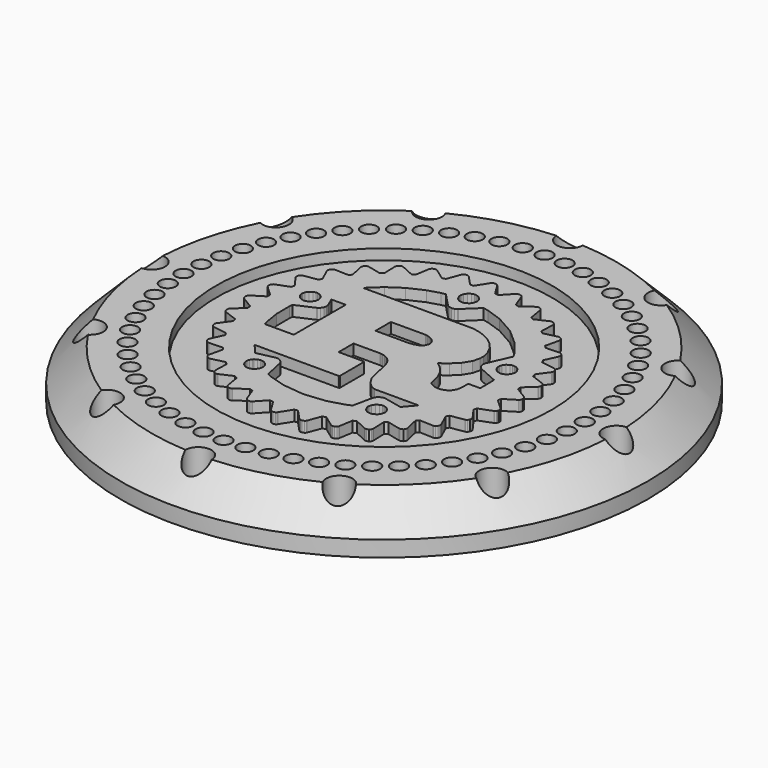
from build123d import *

# Parameters (mm, degrees)
F0_R      = 25
F1_DEPTH  = 3
F2_R      = 0.75
F3_DEPTH  = 3
F4_R      = 1.25
F5_DEPTH  = 3
F7_R      = 15.9136389896
F8_DEPTH  = 1
F10_DEPTH = 1
F11_R     = 25
F11_R_2   = 23
F12_DEPTH = 1.5


# Not quite as in the source:
# - a fillet or chamfer that OpenCascade refuses, or shapes differently, is made with other operations: its cross-section is extruded or revolved along the edge and cut away or added


with BuildPart() as f1:
    # F0 (on Top) → F1 (new body)
    with BuildSketch(Plane.XY):
        Circle(F0_R)
    extrude(amount=F1_DEPTH)

    # F2 (on face) → F3 (cut)
    with BuildSketch(Plane.XY.offset(3)):
        with Locations((0, 19)):
            Circle(F2_R)
        with Locations((-1.9860408021, 18.895916012)):
            Circle(F2_R)
        with Locations((-3.9503221255, 18.5848044139)):
            Circle(F2_R)
        with Locations((-5.8713228931, 18.0700738096)):
            Circle(F2_R)
        with Locations((-7.7279962184, 17.3573636952)):
            Circle(F2_R)
        with Locations((-9.5, 16.4544826719)):
            Circle(F2_R)
        with Locations((-11.1679197936, 15.3713228931)):
            Circle(F2_R)
        with Locations((-12.7134815208, 14.1197516841)):
            Circle(F2_R)
        with Locations((-14.1197516841, 12.7134815208)):
            Circle(F2_R)
        with Locations((-15.3713228931, 11.1679197936)):
            Circle(F2_R)
        with Locations((-16.4544826719, 9.5)):
            Circle(F2_R)
        with Locations((-17.3573636952, 7.7279962184)):
            Circle(F2_R)
        with Locations((-18.0700738096, 5.8713228931)):
            Circle(F2_R)
        with Locations((-18.5848044139, 3.9503221255)):
            Circle(F2_R)
        with Locations((-18.895916012, 1.9860408021)):
            Circle(F2_R)
        with Locations((-19, 0)):
            Circle(F2_R)
        with Locations((-18.895916012, -1.9860408021)):
            Circle(F2_R)
        with Locations((-18.5848044139, -3.9503221255)):
            Circle(F2_R)
        with Locations((-18.0700738096, -5.8713228931)):
            Circle(F2_R)
        with Locations((-17.3573636952, -7.7279962184)):
            Circle(F2_R)
        with Locations((-16.4544826719, -9.5)):
            Circle(F2_R)
        with Locations((-15.3713228931, -11.1679197936)):
            Circle(F2_R)
        with Locations((-14.1197516841, -12.7134815208)):
            Circle(F2_R)
        with Locations((-12.7134815208, -14.1197516841)):
            Circle(F2_R)
        with Locations((-11.1679197936, -15.3713228931)):
            Circle(F2_R)
        with Locations((-9.5, -16.4544826719)):
            Circle(F2_R)
        with Locations((-7.7279962184, -17.3573636952)):
            Circle(F2_R)
        with Locations((-5.8713228931, -18.0700738096)):
            Circle(F2_R)
        with Locations((-3.9503221255, -18.5848044139)):
            Circle(F2_R)
        with Locations((-1.9860408021, -18.895916012)):
            Circle(F2_R)
        with Locations((0, -19)):
            Circle(F2_R)
        with Locations((1.9860408021, -18.895916012)):
            Circle(F2_R)
        with Locations((3.9503221255, -18.5848044139)):
            Circle(F2_R)
        with Locations((5.8713228931, -18.0700738096)):
            Circle(F2_R)
        with Locations((7.7279962184, -17.3573636952)):
            Circle(F2_R)
        with Locations((9.5, -16.4544826719)):
            Circle(F2_R)
        with Locations((11.1679197936, -15.3713228931)):
            Circle(F2_R)
        with Locations((12.7134815208, -14.1197516841)):
            Circle(F2_R)
        with Locations((14.1197516841, -12.7134815208)):
            Circle(F2_R)
        with Locations((15.3713228931, -11.1679197936)):
            Circle(F2_R)
        with Locations((16.4544826719, -9.5)):
            Circle(F2_R)
        with Locations((17.3573636952, -7.7279962184)):
            Circle(F2_R)
        with Locations((18.0700738096, -5.8713228931)):
            Circle(F2_R)
        with Locations((18.5848044139, -3.9503221255)):
            Circle(F2_R)
        with Locations((18.895916012, -1.9860408021)):
            Circle(F2_R)
        with Locations((19, 0)):
            Circle(F2_R)
        with Locations((18.895916012, 1.9860408021)):
            Circle(F2_R)
        with Locations((18.5848044139, 3.9503221255)):
            Circle(F2_R)
        with Locations((18.0700738096, 5.8713228931)):
            Circle(F2_R)
        with Locations((17.3573636952, 7.7279962184)):
            Circle(F2_R)
        with Locations((16.4544826719, 9.5)):
            Circle(F2_R)
        with Locations((15.3713228931, 11.1679197936)):
            Circle(F2_R)
        with Locations((14.1197516841, 12.7134815208)):
            Circle(F2_R)
        with Locations((12.7134815208, 14.1197516841)):
            Circle(F2_R)
        with Locations((11.1679197936, 15.3713228931)):
            Circle(F2_R)
        with Locations((9.5, 16.4544826719)):
            Circle(F2_R)
        with Locations((7.7279962184, 17.3573636952)):
            Circle(F2_R)
        with Locations((5.8713228931, 18.0700738096)):
            Circle(F2_R)
        with Locations((3.9503221255, 18.5848044139)):
            Circle(F2_R)
        with Locations((1.9860408021, 18.895916012)):
            Circle(F2_R)
    extrude(amount=-F3_DEPTH, mode=Mode.SUBTRACT)

    # F4 (on face) → F5 (cut)
    with BuildSketch(Plane.XY.offset(3)):
        with Locations((0, 22)):
            Circle(F4_R)
        with Locations((-11, 19.0525588833)):
            Circle(F4_R)
        with Locations((-19.0525588833, 11)):
            Circle(F4_R)
        with Locations((-22, 0)):
            Circle(F4_R)
        with Locations((-19.0525588833, -11)):
            Circle(F4_R)
        with Locations((-11, -19.0525588833)):
            Circle(F4_R)
        with Locations((0, -22)):
            Circle(F4_R)
        with Locations((11, -19.0525588833)):
            Circle(F4_R)
        with Locations((19.0525588833, -11)):
            Circle(F4_R)
        with Locations((22, 0)):
            Circle(F4_R)
        with Locations((19.0525588833, 11)):
            Circle(F4_R)
        with Locations((11, 19.0525588833)):
            Circle(F4_R)
    extrude(amount=-F5_DEPTH, mode=Mode.SUBTRACT)

    # F6: chamfer of 3 on 1 edges, made by hand

    # F6_s1 → F6_t2 (revolve, cut)
    with BuildSketch(Plane.XZ):
        Polygon((25, 0), (22, 3), (25, 3), align=None)
    revolve(axis=Axis((0, 0, 3), (0, 0, 1)), mode=Mode.SUBTRACT)

    # F7 (on face) → F8 (cut)
    with BuildSketch(Plane.XY.offset(3)):
        Circle(F7_R)
    extrude(amount=-F8_DEPTH, mode=Mode.SUBTRACT)

    # F9 (on face) → F10 (join)
    with BuildSketch(Plane.XY.offset(2)):
        Polygon((12.98642, 0.32225), (11.88072, 1.00693), (11.84932, 1.32865), (12.79912, 2.21461), (12.83232, 2.24554), (12.89522, 2.37737), (12.90122, 2.56567), (12.82412, 2.73707), (12.71512, 2.83417), (12.67332, 2.84937), (11.45912, 3.30347), (11.36372, 3.61707), (12.12162, 4.66957), (12.14762, 4.70647), (12.18402, 4.84757), (12.15302, 5.03307), (12.04342, 5.18607), (11.91822, 5.26037), (11.87362, 5.26747), (10.59332, 5.47577), (10.43912, 5.76337), (10.97732, 6.94447), (10.99582, 6.98557), (11.00452, 7.13157), (10.93832, 7.30797), (10.80112, 7.43697), (10.66332, 7.48417), (10.61822, 7.48267), (9.31832, 7.43697), (9.11322, 7.68657), (9.41162, 8.95237), (9.42192, 8.99687), (9.40132, 9.14117), (9.30152, 9.30057), (9.14252, 9.40047), (8.99822, 9.42057), (8.95432, 9.41017), (7.68862, 9.11187), (7.43902, 9.31697), (7.48452, 10.61687), (7.48622, 10.66237), (7.43792, 10.79967), (7.30872, 10.93647), (7.13302, 11.00367), (6.98702, 10.99547), (6.94632, 10.97657), (5.76522, 10.43787), (5.47772, 10.59237), (5.26882, 11.87337), (5.26182, 11.91787), (5.18742, 12.04307), (5.03442, 12.15227), (4.84892, 12.18367), (4.70782, 12.14727), (4.67152, 12.12077), (3.61842, 11.36337), (3.30542, 11.45787), (2.85132, 12.67257), (2.83552, 12.71537), (2.73842, 12.82437), (2.56647, 12.90147), (2.3782, 12.89607), (2.24745, 12.83257), (2.21654, 12.79947), (1.33058, 11.84837), (1.00884, 11.87987), (0.32418, 12.98557), (0.3003, 13.02407), (0.18365, 13.11197), (0.00027, 13.15377), (-0.1831, 13.11197), (-0.2992, 13.02407), (-0.32253, 12.98557), (-1.00667, 11.87987), (-1.32894, 11.84837), (-2.21544, 12.79947), (-2.24637, 12.83257), (-2.37766, 12.89607), (-2.56591, 12.90147), (-2.73789, 12.82437), (-2.83446, 12.71537), (-2.8502, 12.67257), (-3.3043, 11.45787), (-3.61734, 11.36337), (-4.66987, 12.12077), (-4.70675, 12.14727), (-4.84781, 12.18427), (-5.03337, 12.15287), (-5.18744, 12.04307), (-5.26123, 11.91787), (-5.26828, 11.87337), (-5.47662, 10.59237), (-5.76416, 10.43787), (-6.94525, 10.97657), (-6.98649, 10.99547), (-7.13243, 11.00367), (-7.30821, 10.93697), (-7.43733, 10.79967), (-7.48508, 10.66237), (-7.48345, 10.61687), (-7.43787, 9.31697), (-7.68744, 9.11187), (-8.95317, 9.41017), (-8.99766, 9.42057), (-9.14198, 9.40047), (-9.30148, 9.30007), (-9.40185, 9.14117), (-9.42138, 8.99687), (-9.41107, 8.95237), (-9.11323, 7.68657), (-9.31775, 7.43697), (-10.61767, 7.48267), (-10.66324, 7.48417), (-10.79996, 7.43607), (-10.93669, 7.30687), (-11.00395, 7.13107), (-10.99582, 6.98557), (-10.97682, 6.94447), (-10.43863, 5.76337), (-10.59271, 5.47577), (-11.87364, 5.26747), (-11.91867, 5.26037), (-12.04399, 5.18667), (-12.15251, 5.03307), (-12.18396, 4.84757), (-12.14762, 4.70647), (-12.12103, 4.66957), (-11.36366, 3.61707), (-11.4586, 3.30347), (-12.67334, 2.84937), (-12.71566, 2.83367), (-12.82416, 2.73707), (-12.9012, 2.56567), (-12.89577, 2.37737), (-12.8323, 2.24554), (-12.7992, 2.21461), (-11.84923, 1.32865), (-11.88069, 1.00693), (-12.98584, 0.32225), (-13.02435, 0.29891), (-13.11224, 0.18228), (-13.15402, -0.0011), (-13.11224, -0.18447), (-13.02435, -0.30059), (-12.98584, -0.32445), (-11.88069, -1.00859), (-11.84923, -1.33085), (-12.7992, -2.21735), (-12.8323, -2.24774), (-12.89577, -2.37903), (-12.9012, -2.56675), (-12.82416, -2.73872), (-12.71566, -2.83585), (-12.67334, -2.85157), (-11.4586, -3.30568), (-11.36366, -3.61927), (-12.12103, -4.67178), (-12.14762, -4.70813), (-12.18396, -4.84974), (-12.15251, -5.03528), (-12.04345, -5.18828), (-11.91813, -5.2626), (-11.8731, -5.26966), (-10.59271, -5.47799), (-10.43863, -5.76607), (-10.97682, -6.94663), (-10.99582, -6.98732), (-11.0045, -7.13326), (-10.93723, -7.30904), (-10.79996, -7.43871), (-10.6627, -7.48645), (-10.61767, -7.48482), (-9.3183, -7.43925), (-9.11323, -7.68882), (-9.41107, -8.95509), (-9.42138, -8.9985), (-9.40185, -9.14281), (-9.30148, -9.30232), (-9.14198, -9.4016), (-8.99766, -9.42221), (-8.95317, -9.41191), (-7.68744, -9.11352), (-7.43787, -9.3186), (-7.48345, -10.6185), (-7.48508, -10.66353), (-7.43733, -10.80079), (-7.30821, -10.93752), (-7.13243, -11.00425), (-6.98649, -10.99611), (-6.94525, -10.97767), (-5.76416, -10.43947), (-5.47662, -10.59409), (-5.26828, -11.87393), (-5.26123, -11.91842), (-5.18744, -12.04374), (-5.03337, -12.15279), (-4.84781, -12.18427), (-4.70675, -12.14791), (-4.66987, -12.12186), (-3.61789, -11.36395), (-3.3043, -11.45943), (-2.8502, -12.67363), (-2.83446, -12.71541), (-2.73789, -12.82391), (-2.56591, -12.90095), (-2.3782, -12.89553), (-2.24691, -12.83259), (-2.21598, -12.7995), (-1.32948, -11.84952), (-1.00721, -11.88153), (-0.32253, -12.98721), (-0.2992, -13.0252), (-0.1831, -13.112), (0.00027, -13.15377), (0.18365, -13.11254), (0.3003, -13.0252), (0.32418, -12.98721), (1.0083, -11.88153), (1.33058, -11.84952), (2.21654, -12.7995), (2.24691, -12.83204), (2.3782, -12.89553), (2.56647, -12.90095), (2.73842, -12.82391), (2.83552, -12.71541), (2.85132, -12.67363), (3.30542, -11.45943), (3.61842, -11.36395), (4.67092, -12.12186), (4.70732, -12.14791), (4.84832, -12.18427), (5.03392, -12.15279), (5.18742, -12.04374), (5.26122, -11.91842), (5.26882, -11.87393), (5.47772, -10.59409), (5.76522, -10.43947), (6.94632, -10.97767), (6.98702, -10.99611), (7.13252, -11.00479), (7.30872, -10.93806), (7.43732, -10.80079), (7.48572, -10.66353), (7.48402, -10.6185), (7.43902, -9.3186), (7.68802, -9.11352), (8.95372, -9.41191), (8.99762, -9.42221), (9.14192, -9.4016), (9.30152, -9.30232), (9.40132, -9.14281), (9.42142, -8.9985), (9.41162, -8.95509), (9.11322, -7.68882), (9.31832, -7.43925), (10.61762, -7.48482), (10.66272, -7.48645), (10.80002, -7.43871), (10.93722, -7.30904), (11.00452, -7.13326), (10.99582, -6.98732), (10.97732, -6.94663), (10.43912, -5.76607), (10.59272, -5.47799), (11.87362, -5.26966), (11.91822, -5.2626), (12.04342, -5.18828), (12.15252, -5.03528), (12.18402, -4.84974), (12.14702, -4.70813), (12.12112, -4.67178), (11.36372, -3.61927), (11.45862, -3.30568), (12.67332, -2.85157), (12.71572, -2.83585), (12.82412, -2.73872), (12.90122, -2.56675), (12.89522, -2.37903), (12.83182, -2.24774), (12.79912, -2.21735), (11.84932, -1.33085), (11.88072, -1.00859), (12.98582, -0.32445), (13.02392, -0.30059), (13.11162, -0.18447), (13.15402, -0.0011), (13.11222, 0.18228), (13.02442, 0.29891), align=None)
        Polygon((-6.61593, -8.12068), (-6.61593, -8.04472), (-6.61593, -7.96985), (-6.5568, -7.74524), (-6.42388, -7.52769), (-6.38699, -7.49134), (-6.35064, -7.45444), (-6.13362, -7.32152), (-5.90901, -7.26239), (-5.83414, -7.26239), (-5.75981, -7.26239), (-5.5352, -7.32152), (-5.31819, -7.45444), (-5.2813, -7.49134), (-5.24495, -7.52769), (-5.11203, -7.74524), (-5.05235, -7.96985), (-5.05235, -8.04472), (-5.05235, -8.12068), (-5.1142, -8.34854), (-5.2813, -8.59756), (-5.53032, -8.76466), (-5.75819, -8.82651), (-5.83414, -8.82651), (-5.91064, -8.82651), (-6.1385, -8.76466), (-6.38699, -8.59756), (-6.55463, -8.34854), align=None, mode=Mode.SUBTRACT)
        Polygon((4.96992, -8.15703), (4.96992, -8.08107), (4.96992, -8.00457), (5.03122, -7.77671), (5.19882, -7.52823), (5.44732, -7.36058), (5.67522, -7.29928), (5.75172, -7.29928), (5.82762, -7.29928), (6.05552, -7.36058), (6.30452, -7.52823), (6.47222, -7.77671), (6.53402, -8.00457), (6.53402, -8.08107), (6.53402, -8.15703), (6.47222, -8.38489), (6.30452, -8.63337), (6.05552, -8.80047), (5.82762, -8.86232), (5.75172, -8.86232), (5.67522, -8.86232), (5.44732, -8.80047), (5.19882, -8.63337), (5.03122, -8.38489), align=None, mode=Mode.SUBTRACT)
        Polygon((6.86552, -6.66343), (5.21192, -6.30753), (5.14352, -6.29288), (4.92812, -6.30372), (4.67472, -6.40572), (4.47782, -6.59561), (4.37912, -6.78767), (4.36492, -6.85603), (3.97272, -8.68762), (3.50182, -8.9003), (1.99788, -9.33596), (-0.04584, -9.54538), (-2.08794, -9.31588), (-3.58751, -8.86666), (-4.05571, -8.6491), (-4.44796, -6.81751), (-4.46262, -6.74969), (-4.56135, -6.55763), (-4.7583, -6.36775), (-5.01166, -6.26575), (-5.22705, -6.25491), (-5.29432, -6.26954), (-6.91162, -6.61677), (-6.98703, -6.53919), (-7.68364, -5.71779), (-7.74766, -5.63099), (0.12018, -5.63099), (0.14676, -5.63099), (0.22759, -5.61254), (0.26883, -5.5534), (0.26883, -5.53386), (0.26883, -2.75121), (0.26883, -2.73114), (0.22759, -2.672), (0.14676, -2.6541), (0.12018, -2.6541), (-2.18071, -2.6541), (-2.18071, -0.88977), (0.3079, -0.88977), (0.33719, -0.88977), (0.42562, -0.89465), (0.59815, -0.91961), (0.80865, -0.97657), (1.03977, -1.07965), (1.27523, -1.24188), (1.49768, -1.47679), (1.69081, -1.79743), (1.81126, -2.10939), (1.83838, -2.21681), (1.8628, -2.31393), (1.9317, -2.64488), (2.05161, -3.2384), (2.18127, -3.83465), (2.26536, -4.17047), (2.3028, -4.27193), (2.33697, -4.37664), (2.49213, -4.67559), (2.81332, -5.12154), (3.22732, -5.48234), (3.57772, -5.63099), (3.69492, -5.63099), (7.75692, -5.63099), (7.68862, -5.72213), (6.94582, -6.58259), align=None, mode=Mode.SUBTRACT)
        Polygon((-9.57221, 1.11815), (-7.88764, 1.86684), (-7.8247, 1.89505), (-7.65706, 2.03069), (-7.51166, 2.26236), (-7.46392, 2.53197), (-7.49755, 2.74517), (-7.52522, 2.80867), (-7.8719, 3.59317), (-6.50743, 3.59317), (-6.50743, -2.55699), (-9.26026, -2.55699), (-9.34542, -2.25859), (-9.59391, -0.73407), (-9.60584, 0.80998), align=None, mode=Mode.SUBTRACT)
        Polygon((-10.15109, 2.89817), (-10.15109, 2.97417), (-10.15109, 3.05067), (-10.08978, 3.27857), (-9.92214, 3.52697), (-9.67366, 3.69467), (-9.4458, 3.75597), (-9.3693, 3.75597), (-9.29334, 3.75597), (-9.06548, 3.69467), (-8.81645, 3.52697), (-8.64935, 3.27857), (-8.58751, 3.05067), (-8.58751, 2.97417), (-8.58751, 2.89817), (-8.64935, 2.67037), (-8.81645, 2.42187), (-9.06548, 2.25422), (-9.29334, 2.19237), (-9.3693, 2.19237), (-9.4458, 2.19237), (-9.67366, 2.25422), (-9.92214, 2.42187), (-10.08978, 2.67037), align=None, mode=Mode.SUBTRACT)
        Polygon((-0.82275, 9.97827), (-0.82275, 10.05427), (-0.82275, 10.13077), (-0.76144, 10.35867), (-0.5938, 10.60717), (-0.34532, 10.77477), (-0.11745, 10.83607), (-0.04095, 10.83607), (0.03499, 10.83607), (0.26287, 10.77477), (0.51188, 10.60717), (0.67898, 10.35867), (0.74084, 10.13077), (0.74084, 10.05427), (0.74084, 9.97827), (0.67898, 9.75047), (0.51188, 9.50147), (0.26287, 9.33437), (0.03499, 9.27237), (-0.04095, 9.27237), (-0.11745, 9.27237), (-0.34532, 9.33437), (-0.5938, 9.50147), (-0.76144, 9.75047), align=None, mode=Mode.SUBTRACT)
        Polygon((0.83198, 1.71548), (-2.18017, 1.71548), (-2.18017, 3.52807), (1.06852, 3.52807), (1.09294, 3.52807), (1.16727, 3.51827), (1.32461, 3.48627), (1.5172, 3.42717), (1.72391, 3.33657), (1.92302, 3.21017), (2.09229, 3.04417), (2.20948, 2.83367), (2.25397, 2.63887), (2.25397, 2.57377), (2.25397, 2.47397), (2.12159, 2.17337), (1.78359, 1.90808), (1.32461, 1.76105), (0.95513, 1.71548), align=None, mode=Mode.SUBTRACT)
        Polygon((7.80472, 1.82887), (9.58042, 1.04057), (9.59392, 0.90168), (9.61122, -0.49156), (9.60092, -0.63099), (8.61302, -0.63099), (8.58642, -0.63099), (8.50662, -0.67493), (8.47472, -0.76282), (8.47472, -0.79266), (8.47472, -1.24622), (8.47472, -1.40952), (8.37202, -1.90052), (8.10732, -2.30361), (7.74392, -2.51792), (7.44552, -2.59388), (7.34512, -2.60527), (7.25182, -2.61557), (6.96642, -2.59116), (6.61822, -2.4832), (6.35122, -2.30634), (6.22962, -2.14682), (6.21662, -2.08768), (6.17002, -1.82672), (5.95572, -1.0585), (5.61282, -0.37382), (5.17932, 0.11337), (4.78162, 0.44432), (4.64652, 0.55065), (4.83262, 0.66893), (5.36322, 1.06715), (5.99692, 1.69378), (6.44882, 2.43267), (6.62142, 3.07237), (6.62142, 3.28557), (6.62142, 3.50907), (6.47112, 4.17917), (6.09562, 4.89577), (5.60462, 5.44327), (5.24062, 5.74057), (5.11092, 5.82627), (4.95792, 5.92717), (4.46102, 6.17187), (3.85122, 6.37857), (3.35422, 6.48007), (3.12152, 6.50607), (3.04392, 6.50607), (-7.17149, 6.50607), (-6.90944, 6.79907), (-6.02728, 7.59177), (-4.72955, 8.47057), (-3.30648, 9.12697), (-2.17203, 9.47327), (-1.78574, 9.54587), (-0.58132, 8.28287), (-0.53357, 8.23297), (-0.34912, 8.12057), (-0.08219, 8.06197), (0.18691, 8.10807), (0.37626, 8.21187), (0.4267, 8.25947), (1.77383, 9.54807), (2.28544, 9.45257), (3.77902, 8.94107), (5.58572, 7.92757), (7.13452, 6.55107), (8.10622, 5.30647), (8.36452, 4.85407), (7.44222, 2.77127), (7.41402, 2.70777), (7.38092, 2.49457), (7.42872, 2.22491), (7.57402, 1.99326), (7.74122, 1.85708), align=None, mode=Mode.SUBTRACT)
        Polygon((8.50512, 2.86187), (8.50512, 2.93777), (8.50512, 3.01427), (8.56632, 3.24217), (8.73402, 3.49067), (8.98252, 3.65827), (9.21042, 3.71957), (9.28682, 3.71957), (9.36272, 3.71957), (9.59072, 3.65827), (9.83972, 3.49067), (10.00682, 3.24217), (10.06862, 3.01427), (10.06862, 2.93777), (10.06862, 2.86187), (10.00682, 2.63397), (9.83972, 2.38547), (9.59072, 2.21841), (9.36272, 2.15655), (9.28682, 2.15655), (9.21042, 2.15655), (8.98252, 2.21841), (8.73402, 2.38547), (8.56632, 2.63397), align=None, mode=Mode.SUBTRACT)
    extrude(amount=F10_DEPTH)

    # F11 (on face) → F12 (join)
    with BuildSketch(Plane(origin=(0, 0, 0), x_dir=(1, 0, 0), z_dir=(0, 0, -1))):
        Circle(F11_R)
        Circle(F11_R_2, mode=Mode.SUBTRACT)
    extrude(amount=F12_DEPTH)


solid = f1.part
